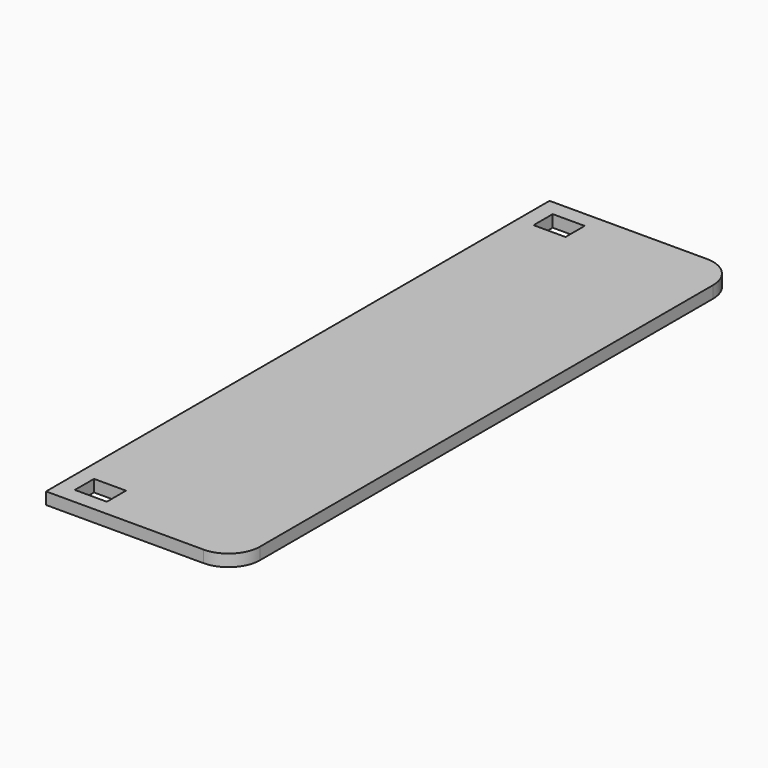
from build123d import *

# Parameters (mm, degrees)
F0_W     = 300
F0_H     = 1000
F1_DEPTH = 19.05
F2_W     = 50.8
F2_H     = 38.1
F3_DEPTH = 19.05
F4_R     = 50


# Not quite as in the source:
# - a length typed as a fraction of an inch, garbled in the dataset ("3 / 203.2 mm" for 3/8 in), is restored


with BuildPart() as f1:
    # F0 (on Top) → F1 (new body)
    with BuildSketch(Plane.XY):
        with Locations((150, 500)):
            Rectangle(F0_W, F0_H)
    extrude(amount=F1_DEPTH)

    # F2 (on face) → F3 (cut, through all)
    with BuildSketch(Plane.XY.offset(19.05)):
        with Locations((50.8, 44.45)):
            Rectangle(F2_W, F2_H)
        with Locations((50.8, 955.55)):
            Rectangle(F2_W, F2_H)
    extrude(amount=-F3_DEPTH, mode=Mode.SUBTRACT)

    # F4
    f4_edges = [f1.edges().sort_by_distance(p)[0] for p in [
        (300, 0, 9.525),
        (300, 1000, 9.525),
    ]]
    fillet(f4_edges, radius=F4_R)


solid = f1.part
